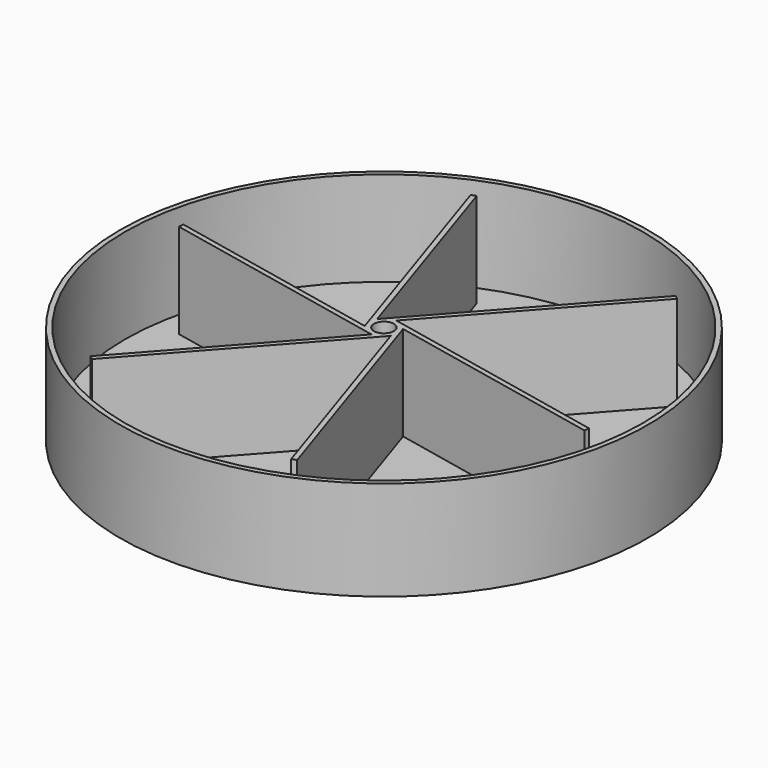
from build123d import *

# Parameters (mm, degrees)
F4_DEPTH        = 60.325
F4_COPIES_COUNT = 6


# Not quite as in the source:
# - a pattern or mirror of a feature is missing from the dataset's text; its kind, count and spacing are read off the source's solid


with BuildPart() as f2:
    # F0 (on Front) → F2 (revolve)
    with BuildSketch(Plane.XZ):
        Polygon((-9.525, 0), (-6.35, 0), (-6.35, 63.5), (-9.525, 63.5), (-9.525, 38.1), (-9.525, 3.175), (-18.9311246582, 3.175), (-139.6226100799, 3.175), (-165.1, 3.175), (-165.1, 38.1), (-165.1, 63.5), (-168.275, 63.5), (-168.275, 0), (-165.1, 0), (-139.7, 0), (-19.05, 0), align=None)
    revolve(axis=Axis((0, 0, 2.6372056454), (0, 0, -1)))

    # F3 (on face) → F4 (join, through all)
    with BuildSketch(Plane.XY.offset(63.5)):
        with BuildLine():
            Line((-92.1809510877, -117.3489364313), (7.0995158286, -6.35))
            ThreePointArc((7.0995158286, -6.35), (3.8885649667, -8.6950956004), (0, -9.525))
            Line((0, -9.525), (-94.6602110475, -115.3583333333))
            ThreePointArc((-94.6602110475, -115.3583333333), (-93.4258828815, -116.3602381951), (-92.1809510877, -117.3489364313))
        make_face()
    f4 = extrude(amount=-F4_DEPTH)

    # F4_copies: F4 ×6 about axis
    f4_copies_axis = Axis((0, 0, 0), (0, 0, 1))
    for i in range(1, F4_COPIES_COUNT):
        add(f4.rotate(f4_copies_axis, i * 360 / F4_COPIES_COUNT))


solid = f2.part
